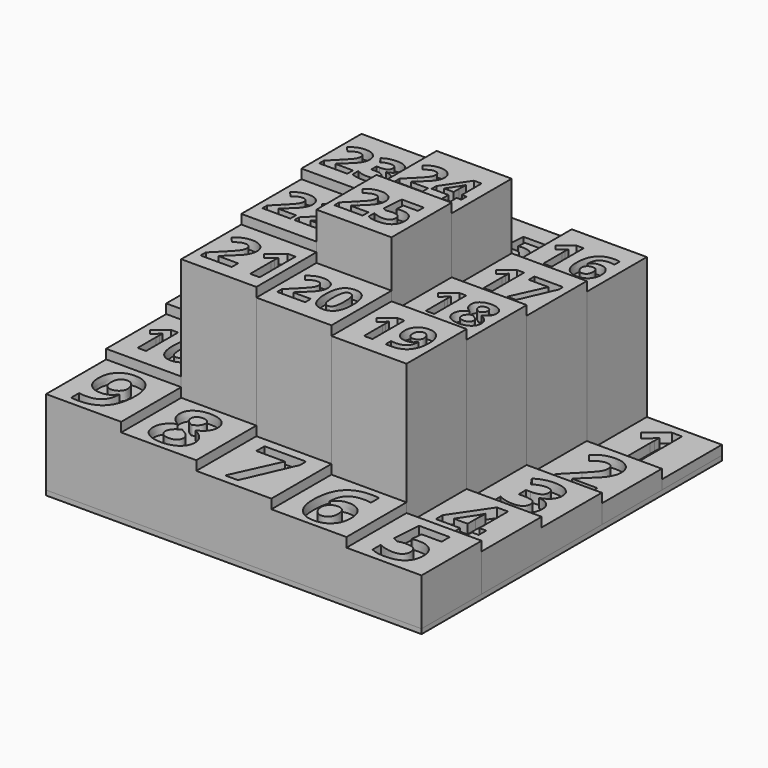
from build123d import *

# Parameters (mm, degrees)
F0_W          = 40
F0_H          = 40
F1_DEPTH      = 5
F2_W          = 40
F2_H          = 40
F3_DEPTH      = 10
F4_W          = 40
F4_H          = 40
F5_DEPTH      = 15
F6_W          = 40
F6_H          = 40
F7_DEPTH      = 20
F8_W          = 40
F8_H          = 40
F9_DEPTH      = 25
F10_W         = 40
F10_H         = 40
F11_DEPTH     = 30
F12_W         = 40
F12_H         = 40
F13_DEPTH     = 35
F14_W         = 40
F14_H         = 40
F15_DEPTH     = 40
F16_W         = 40
F16_H         = 40
F17_DEPTH     = 45
F18_W         = 40
F18_H         = 40
F19_DEPTH     = 50
F20_W         = 40
F20_H         = 40
F21_DEPTH     = 55
F22_W         = 40
F22_H         = 40
F23_DEPTH     = 60
F24_W         = 40
F24_H         = 40
F25_DEPTH     = 65
F26_W         = 40
F26_H         = 40
F27_DEPTH     = 70
F28_W         = 40
F28_H         = 40
F29_DEPTH     = 75
F30_W         = 40
F30_H         = 40
F31_DEPTH     = 80
F32_W         = 40
F32_H         = 40
F33_DEPTH     = 85
F34_W         = 40
F34_H         = 40
F35_DEPTH     = 90
F36_W         = 40
F36_H         = 40
F37_DEPTH     = 95
F38_W         = 40
F38_H         = 40
F39_DEPTH     = 100
F40_W         = 40
F40_H         = 40
F41_DEPTH     = 105
F42_W         = 40
F42_H         = 40
F43_DEPTH     = 110
F44_W         = 40
F44_H         = 40
F45_DEPTH     = 115
F46_W         = 40
F46_H         = 40
F47_DEPTH     = 120
F48_W         = 40
F48_H         = 40
F49_DEPTH     = 125
F50_TEXT_SIZE = 43.9635064039
F51_DEPTH     = 25.4
F52_TEXT_SIZE = 42.8115716204
F53_DEPTH     = 5
F54_TEXT_SIZE = 41.7113808605
F55_DEPTH     = 5
F56_TEXT_SIZE = 42.539030417
F57_DEPTH     = 5
F58_TEXT_SIZE = 42.0912582841
F59_DEPTH     = 5
F60_TEXT_SIZE = 45.2257071932
F61_DEPTH     = 5
F62_TEXT_SIZE = 43.1709095008
F63_DEPTH     = 5
F64_TEXT_SIZE = 44.5941256152
F65_DEPTH     = 5
F66_TEXT_SIZE = 44.0766827928
F67_DEPTH     = 5
F68_TEXT_SIZE = 29.8945682637
F69_DEPTH     = 5
F70_TEXT_SIZE = 33.3730631704
F71_DEPTH     = 5
F72_TEXT_SIZE = 29.7951582868
F73_DEPTH     = 5
F74_TEXT_SIZE = 29.970564624
F75_DEPTH     = 5
F76_TEXT_SIZE = 29.39246818
F77_DEPTH     = 5
F78_TEXT_SIZE = 30.131826742
F79_DEPTH     = 5
F80_TEXT_SIZE = 29.7951582868
F81_DEPTH     = 5
F82_TEXT_SIZE = 29.7951582868
F83_DEPTH     = 5
F84_TEXT_SIZE = 29.8706494199
F85_DEPTH     = 5
F86_TEXT_SIZE = 29.8706494199
F87_DEPTH     = 5
F88_TEXT_SIZE = 29.8945682637
F89_DEPTH     = 5
F90_TEXT_SIZE = 33.3730631704
F91_DEPTH     = 5
F92_TEXT_SIZE = 29.7951582868
F93_DEPTH     = 5
F94_TEXT_SIZE = 29.970564624
F95_DEPTH     = 5
F96_TEXT_SIZE = 29.39246818
F97_DEPTH     = 5
F98_TEXT_SIZE = 30.131826742
F99_DEPTH     = 5
F101_ANGLE    = 180
F102_W        = 200
F102_H        = 200
F103_DEPTH    = 2.54


# Not quite as in the source:
# - Text() gives the source's letters only with a copy of the font that has no kerning and outlines rounded to 1/6400 em; it was checked with that copy


with BuildPart() as f1:
    # F0 (on Top) → F1 (new body)
    with BuildSketch(Plane.XY):
        with Locations((-146.1425478756, 78.8295151293)):
            Rectangle(F0_W, F0_H)
    extrude(amount=F1_DEPTH)

    # F50 (on face) → F51 (cut)
    with BuildSketch(Plane.XY.offset(5)):
        with Locations((-161.8985384703, 62.9098713398)):
            Text('1', F50_TEXT_SIZE, font='Open Sans', font_style=FontStyle.BOLD, text_align=(TextAlign.LEFT, TextAlign.BOTTOM))
    extrude(amount=-F51_DEPTH, mode=Mode.SUBTRACT)


with BuildPart() as f3:
    # F2 (on face) → F3 (new body)
    with BuildSketch(Plane(origin=(0, 0, 0), x_dir=(1, 0, 0), z_dir=(0, 0, -1))):
        with Locations((-146.1425478756, -38.8295151293)):
            Rectangle(F2_W, F2_H)
    extrude(amount=-F3_DEPTH)

    # F52 (on face) → F53 (cut)
    with BuildSketch(Plane.XY.offset(10)):
        with Locations((-159.3360304832, 23.0267103761)):
            Text('2', F52_TEXT_SIZE, font='Open Sans', font_style=FontStyle.BOLD, text_align=(TextAlign.LEFT, TextAlign.BOTTOM))
    extrude(amount=-F53_DEPTH, mode=Mode.SUBTRACT)


with BuildPart() as f5:
    # F4 (on face) → F5 (new body)
    with BuildSketch(Plane(origin=(0, 0, 0), x_dir=(1, 0, 0), z_dir=(0, 0, -1))):
        with Locations((-146.1425478756, 1.1704848707)):
            Rectangle(F4_W, F4_H)
    extrude(amount=-F5_DEPTH)

    # F6 (on face) → F7 (join)
    with BuildSketch(Plane(origin=(0, 0, 0), x_dir=(1, 0, 0), z_dir=(0, 0, -1))):
        with Locations((-146.1425478756, 41.1704848707)):
            Rectangle(F6_W, F6_H)
    extrude(amount=-F7_DEPTH)

    # F54 (on face) → F55 (cut)
    with BuildSketch(Plane.XY.offset(15)):
        with Locations((-158.4442704916, -16.6733469814)):
            Text('3', F54_TEXT_SIZE, font='Open Sans', font_style=FontStyle.BOLD, text_align=(TextAlign.LEFT, TextAlign.BOTTOM))
    extrude(amount=-F55_DEPTH, mode=Mode.SUBTRACT)

    # F56 (on face) → F57 (cut)
    with BuildSketch(Plane.XY.offset(20)):
        with Locations((-159.9645316601, -56.619418785)):
            Text('4', F56_TEXT_SIZE, font='Open Sans', font_style=FontStyle.BOLD, text_align=(TextAlign.LEFT, TextAlign.BOTTOM))
    extrude(amount=-F57_DEPTH, mode=Mode.SUBTRACT)


with BuildPart() as f9:
    # F8 (on face) → F9 (new body)
    with BuildSketch(Plane(origin=(0, 0, 0), x_dir=(1, 0, 0), z_dir=(0, 0, -1))):
        with Locations((-146.1425478756, 81.1704848707)):
            Rectangle(F8_W, F8_H)
    extrude(amount=-F9_DEPTH)

    # F10 (on face) → F11 (join)
    with BuildSketch(Plane(origin=(0, 0, 0), x_dir=(1, 0, 0), z_dir=(0, 0, -1))):
        with Locations((-186.1425478756, 81.1704848707)):
            Rectangle(F10_W, F10_H)
    extrude(amount=-F11_DEPTH)

    # F12 (on face) → F13 (join)
    with BuildSketch(Plane(origin=(0, 0, 0), x_dir=(1, 0, 0), z_dir=(0, 0, -1))):
        with Locations((-226.1425478756, 81.1704848707)):
            Rectangle(F12_W, F12_H)
    extrude(amount=-F13_DEPTH)

    # F14 (on face) → F15 (join)
    with BuildSketch(Plane(origin=(0, 0, 0), x_dir=(1, 0, 0), z_dir=(0, 0, -1))):
        with Locations((-266.1425478756, 81.1704848707)):
            Rectangle(F14_W, F14_H)
    extrude(amount=-F15_DEPTH)

    # F16 (on face) → F17 (join)
    with BuildSketch(Plane(origin=(0, 0, 0), x_dir=(1, 0, 0), z_dir=(0, 0, -1))):
        with Locations((-306.1425478756, 81.1704848707)):
            Rectangle(F16_W, F16_H)
    extrude(amount=-F17_DEPTH)

    # F18 (on face) → F19 (join)
    with BuildSketch(Plane(origin=(0, 0, 0), x_dir=(1, 0, 0), z_dir=(0, 0, -1))):
        with Locations((-306.1425478756, 41.1704848707)):
            Rectangle(F18_W, F18_H)
    extrude(amount=-F19_DEPTH)

    # F20 (on face) → F21 (join)
    with BuildSketch(Plane(origin=(0, 0, 0), x_dir=(1, 0, 0), z_dir=(0, 0, -1))):
        with Locations((-306.1425478756, 1.1704848707)):
            Rectangle(F20_W, F20_H)
    extrude(amount=-F21_DEPTH)

    # F22 (on face) → F23 (join)
    with BuildSketch(Plane(origin=(0, 0, 0), x_dir=(1, 0, 0), z_dir=(0, 0, -1))):
        with Locations((-306.1425478756, -38.8295151293)):
            Rectangle(F22_W, F22_H)
    extrude(amount=-F23_DEPTH)

    # F58 (on face) → F59 (cut)
    with BuildSketch(Plane.XY.offset(25)):
        with Locations((-158.6749255657, -96.9195589423)):
            Text('5', F58_TEXT_SIZE, font='Open Sans', font_style=FontStyle.BOLD, text_align=(TextAlign.LEFT, TextAlign.BOTTOM))
    extrude(amount=-F59_DEPTH, mode=Mode.SUBTRACT)

    # F60 (on face) → F61 (cut)
    with BuildSketch(Plane.XY.offset(30)):
        with Locations((-199.6198743582, -97.5643545389)):
            Text('6', F60_TEXT_SIZE, font='Open Sans', font_style=FontStyle.BOLD, text_align=(TextAlign.LEFT, TextAlign.BOTTOM))
    extrude(amount=-F61_DEPTH, mode=Mode.SUBTRACT)

    # F62 (on face) → F63 (cut)
    with BuildSketch(Plane.XY.offset(35)):
        with Locations((-239.0029877424, -96.8608111143)):
            Text('7', F62_TEXT_SIZE, font='Open Sans', font_style=FontStyle.BOLD, text_align=(TextAlign.LEFT, TextAlign.BOTTOM))
    extrude(amount=-F63_DEPTH, mode=Mode.SUBTRACT)

    # F64 (on face) → F65 (cut)
    with BuildSketch(Plane.XY.offset(40)):
        with Locations((-280.3331911564, -97.2023829818)):
            Text('8', F64_TEXT_SIZE, font='Open Sans', font_style=FontStyle.BOLD, text_align=(TextAlign.LEFT, TextAlign.BOTTOM))
    extrude(amount=-F65_DEPTH, mode=Mode.SUBTRACT)

    # F66 (on face) → F67 (cut)
    with BuildSketch(Plane.XY.offset(45)):
        with Locations((-319.6105360985, -97.0161855221)):
            Text('9', F66_TEXT_SIZE, font='Open Sans', font_style=FontStyle.BOLD, text_align=(TextAlign.LEFT, TextAlign.BOTTOM))
    extrude(amount=-F67_DEPTH, mode=Mode.SUBTRACT)

    # F68 (on face) → F69 (cut)
    with BuildSketch(Plane.XY.offset(50)):
        with Locations((-324.2531219047, -52.3943256904)):
            Text('10', F68_TEXT_SIZE, font='Open Sans', font_style=FontStyle.BOLD, text_align=(TextAlign.LEFT, TextAlign.BOTTOM))
    extrude(amount=-F69_DEPTH, mode=Mode.SUBTRACT)

    # F70 (on face) → F71 (cut)
    with BuildSketch(Plane.XY.offset(55)):
        with Locations((-323.840325339, -13.2019839741)):
            Text('11', F70_TEXT_SIZE, font='Open Sans', font_style=FontStyle.BOLD, text_align=(TextAlign.LEFT, TextAlign.BOTTOM))
    extrude(amount=-F71_DEPTH, mode=Mode.SUBTRACT)

    # F72 (on face) → F73 (cut)
    with BuildSketch(Plane.XY.offset(60)):
        with Locations((-324.2819103489, 26.9366578012)):
            Text('12', F72_TEXT_SIZE, font='Open Sans', font_style=FontStyle.BOLD, text_align=(TextAlign.LEFT, TextAlign.BOTTOM))
    extrude(amount=-F73_DEPTH, mode=Mode.SUBTRACT)


with BuildPart() as f25:
    # F24 (on face) → F25 (new body)
    with BuildSketch(Plane(origin=(0, 0, 0), x_dir=(1, 0, 0), z_dir=(0, 0, -1))):
        with Locations((-306.1425478756, -78.8295151293)):
            Rectangle(F24_W, F24_H)
    extrude(amount=-F25_DEPTH)

    # F26 (on face) → F27 (join)
    with BuildSketch(Plane(origin=(0, 0, 0), x_dir=(1, 0, 0), z_dir=(0, 0, -1))):
        with Locations((-266.1425478756, -78.8295151293)):
            Rectangle(F26_W, F26_H)
    extrude(amount=-F27_DEPTH)

    # F74 (on face) → F75 (cut)
    with BuildSketch(Plane.XY.offset(65)):
        with Locations((-323.570565288, 67.1331060173)):
            Text('13', F74_TEXT_SIZE, font='Open Sans', font_style=FontStyle.BOLD, text_align=(TextAlign.LEFT, TextAlign.BOTTOM))
    extrude(amount=-F75_DEPTH, mode=Mode.SUBTRACT)

    # F76 (on face) → F77 (cut)
    with BuildSketch(Plane.XY.offset(70)):
        with Locations((-283.8859129857, 67.584938816)):
            Text('14', F76_TEXT_SIZE, font='Open Sans', font_style=FontStyle.BOLD, text_align=(TextAlign.LEFT, TextAlign.BOTTOM))
    extrude(amount=-F77_DEPTH, mode=Mode.SUBTRACT)


with BuildPart() as f29:
    # F28 (on face) → F29 (new body)
    with BuildSketch(Plane(origin=(0, 0, 0), x_dir=(1, 0, 0), z_dir=(0, 0, -1))):
        with Locations((-226.1425478756, -78.8295151293)):
            Rectangle(F28_W, F28_H)
    extrude(amount=-F29_DEPTH)

    # F78 (on face) → F79 (cut)
    with BuildSketch(Plane.XY.offset(75)):
        with Locations((-243.567291904, 67.0035963744)):
            Text('15', F78_TEXT_SIZE, font='Open Sans', font_style=FontStyle.BOLD, text_align=(TextAlign.LEFT, TextAlign.BOTTOM))
    extrude(amount=-F79_DEPTH, mode=Mode.SUBTRACT)


with BuildPart() as f31:
    # F30 (on face) → F31 (new body)
    with BuildSketch(Plane(origin=(0, 0, 0), x_dir=(1, 0, 0), z_dir=(0, 0, -1))):
        with Locations((-186.1425478756, -78.8295151293)):
            Rectangle(F30_W, F30_H)
    extrude(amount=-F31_DEPTH)

    # F80 (on face) → F81 (cut)
    with BuildSketch(Plane.XY.offset(80)):
        with Locations((-203.9077669813, 67.3344114036)):
            Text('16', F80_TEXT_SIZE, font='Open Sans', font_style=FontStyle.BOLD, text_align=(TextAlign.LEFT, TextAlign.BOTTOM))
    extrude(amount=-F81_DEPTH, mode=Mode.SUBTRACT)


with BuildPart() as f33:
    # F32 (on face) → F33 (new body)
    with BuildSketch(Plane(origin=(0, 0, 0), x_dir=(1, 0, 0), z_dir=(0, 0, -1))):
        with Locations((-186.1425478756, -38.8295151293)):
            Rectangle(F32_W, F32_H)
    extrude(amount=-F33_DEPTH)

    # F82 (on face) → F83 (cut)
    with BuildSketch(Plane.XY.offset(85)):
        with Locations((-203.5129799515, 27.1933717301)):
            Text('17', F82_TEXT_SIZE, font='Open Sans', font_style=FontStyle.BOLD, text_align=(TextAlign.LEFT, TextAlign.BOTTOM))
    extrude(amount=-F83_DEPTH, mode=Mode.SUBTRACT)


with BuildPart() as f35:
    # F34 (on face) → F35 (new body)
    with BuildSketch(Plane(origin=(0, 0, 0), x_dir=(1, 0, 0), z_dir=(0, 0, -1))):
        with Locations((-186.1425478756, 1.1704848707)):
            Rectangle(F34_W, F34_H)
    extrude(amount=-F35_DEPTH)

    # F84 (on face) → F85 (cut)
    with BuildSketch(Plane.XY.offset(90)):
        with Locations((-203.4901118982, -11.471883155)):
            Text('18', F84_TEXT_SIZE, font='Open Sans', font_style=FontStyle.BOLD, text_align=(TextAlign.LEFT, TextAlign.BOTTOM))
    extrude(amount=-F85_DEPTH, mode=Mode.SUBTRACT)


with BuildPart() as f37:
    # F36 (on face) → F37 (new body)
    with BuildSketch(Plane(origin=(0, 0, 0), x_dir=(1, 0, 0), z_dir=(0, 0, -1))):
        with Locations((-186.1425478756, 41.1704848707)):
            Rectangle(F36_W, F36_H)
    extrude(amount=-F37_DEPTH)

    # F86 (on face) → F87 (cut)
    with BuildSketch(Plane.XY.offset(95)):
        with Locations((-203.4383152363, -52.6618594744)):
            Text('19', F86_TEXT_SIZE, font='Open Sans', font_style=FontStyle.BOLD, text_align=(TextAlign.LEFT, TextAlign.BOTTOM))
    extrude(amount=-F87_DEPTH, mode=Mode.SUBTRACT)


with BuildPart() as f39:
    # F38 (on face) → F39 (new body)
    with BuildSketch(Plane(origin=(0, 0, 0), x_dir=(1, 0, 0), z_dir=(0, 0, -1))):
        with Locations((-226.1425478756, 41.1704848707)):
            Rectangle(F38_W, F38_H)
    extrude(amount=-F39_DEPTH)

    # F88 (on face) → F89 (cut)
    with BuildSketch(Plane.XY.offset(100)):
        with Locations((-243.8220114889, -51.7340404507)):
            Text('20', F88_TEXT_SIZE, font='Open Sans', font_style=FontStyle.BOLD, text_align=(TextAlign.LEFT, TextAlign.BOTTOM))
    extrude(amount=-F89_DEPTH, mode=Mode.SUBTRACT)


with BuildPart() as f41:
    # F40 (on face) → F41 (new body)
    with BuildSketch(Plane(origin=(0, 0, 0), x_dir=(1, 0, 0), z_dir=(0, 0, -1))):
        with Locations((-266.1425478756, 41.1704848707)):
            Rectangle(F40_W, F40_H)
    extrude(amount=-F41_DEPTH)

    # F90 (on face) → F91 (cut)
    with BuildSketch(Plane.XY.offset(105)):
        with Locations((-283.3203628548, -53.5402236553)):
            Text('21', F90_TEXT_SIZE, font='Open Sans', font_style=FontStyle.BOLD, text_align=(TextAlign.LEFT, TextAlign.BOTTOM))
    extrude(amount=-F91_DEPTH, mode=Mode.SUBTRACT)


with BuildPart() as f43:
    # F42 (on face) → F43 (new body)
    with BuildSketch(Plane(origin=(0, 0, 0), x_dir=(1, 0, 0), z_dir=(0, 0, -1))):
        with Locations((-266.1425478756, 1.1704848707)):
            Rectangle(F42_W, F42_H)
    extrude(amount=-F43_DEPTH)

    # F92 (on face) → F93 (cut)
    with BuildSketch(Plane.XY.offset(110)):
        with Locations((-283.6582310562, -11.7253012178)):
            Text('22', F92_TEXT_SIZE, font='Open Sans', font_style=FontStyle.BOLD, text_align=(TextAlign.LEFT, TextAlign.BOTTOM))
    extrude(amount=-F93_DEPTH, mode=Mode.SUBTRACT)


with BuildPart() as f45:
    # F44 (on face) → F45 (new body)
    with BuildSketch(Plane(origin=(0, 0, 0), x_dir=(1, 0, 0), z_dir=(0, 0, -1))):
        with Locations((-266.1425478756, -38.8295151293)):
            Rectangle(F44_W, F44_H)
    extrude(amount=-F45_DEPTH)

    # F94 (on face) → F95 (cut)
    with BuildSketch(Plane.XY.offset(115)):
        with Locations((-284.4813337052, 27.1075663503)):
            Text('23', F94_TEXT_SIZE, font='Open Sans', font_style=FontStyle.BOLD, text_align=(TextAlign.LEFT, TextAlign.BOTTOM))
    extrude(amount=-F95_DEPTH, mode=Mode.SUBTRACT)


with BuildPart() as f47:
    # F46 (on face) → F47 (new body)
    with BuildSketch(Plane(origin=(0, 0, 0), x_dir=(1, 0, 0), z_dir=(0, 0, -1))):
        with Locations((-226.1425478756, -38.8295151293)):
            Rectangle(F46_W, F46_H)
    extrude(amount=-F47_DEPTH)

    # F96 (on face) → F97 (cut)
    with BuildSketch(Plane.XY.offset(120)):
        with Locations((-243.7350419265, 26.6086359017)):
            Text('24', F96_TEXT_SIZE, font='Open Sans', font_style=FontStyle.BOLD, text_align=(TextAlign.LEFT, TextAlign.BOTTOM))
    extrude(amount=-F97_DEPTH, mode=Mode.SUBTRACT)


with BuildPart() as f49:
    # F48 (on face) → F49 (new body)
    with BuildSketch(Plane(origin=(0, 0, 0), x_dir=(1, 0, 0), z_dir=(0, 0, -1))):
        with Locations((-226.1425478756, 1.1704848707)):
            Rectangle(F48_W, F48_H)
    extrude(amount=-F49_DEPTH)

    # F98 (on face) → F99 (cut)
    with BuildSketch(Plane.XY.offset(125)):
        with Locations((-244.0136139392, -13.3618008085)):
            Text('25', F98_TEXT_SIZE, font='Open Sans', font_style=FontStyle.BOLD, text_align=(TextAlign.LEFT, TextAlign.BOTTOM))
    extrude(amount=-F99_DEPTH, mode=Mode.SUBTRACT)


with BuildPart() as f101_tool:
    # F100 (on face) → F101 (revolve)
    with BuildSketch(Plane(origin=(0, 0, 0), x_dir=(1, 0, 0), z_dir=(0, 0, -1))):
        with BuildLine():
            Line((-225.389104759, 21.1704848707), (-225.389104759, 57.2701077139))
            ThreePointArc((-225.389104759, 57.2701077139), (-282.2472300304, 1.1704848707), (-225.389104759, -54.9291379726))
            Line((-225.389104759, -54.9291379726), (-225.389104759, -18.8295151293))
            Line((-225.389104759, -18.8295151293), (-246.1425478756, -18.8295151293))
            Line((-246.1425478756, -18.8295151293), (-246.1425478756, 21.1704848707))
            Line((-246.1425478756, 21.1704848707), (-225.389104759, 21.1704848707))
        make_face()
    revolve(axis=Axis((-225.389104759, -1.1704848707, 0), (0, 1, 0)), revolution_arc=F101_ANGLE)


with BuildPart() as f33_1:
    add(f33.part)

    # F101: cut by f101_tool
    add(f101_tool.part, mode=Mode.SUBTRACT)


with BuildPart() as f35_1:
    add(f35.part)

    # F101: cut by f101_tool
    add(f101_tool.part, mode=Mode.SUBTRACT)


with BuildPart() as f37_1:
    add(f37.part)

    # F101: cut by f101_tool
    add(f101_tool.part, mode=Mode.SUBTRACT)


with BuildPart() as f39_1:
    add(f39.part)

    # F101: cut by f101_tool
    add(f101_tool.part, mode=Mode.SUBTRACT)


with BuildPart() as f41_1:
    add(f41.part)

    # F101: cut by f101_tool
    add(f101_tool.part, mode=Mode.SUBTRACT)


with BuildPart() as f43_1:
    add(f43.part)

    # F101: cut by f101_tool
    add(f101_tool.part, mode=Mode.SUBTRACT)


with BuildPart() as f45_1:
    add(f45.part)

    # F101: cut by f101_tool
    add(f101_tool.part, mode=Mode.SUBTRACT)


with BuildPart() as f47_1:
    add(f47.part)

    # F101: cut by f101_tool
    add(f101_tool.part, mode=Mode.SUBTRACT)


with BuildPart() as f103:
    # F102 (on face) → F103 (new body)
    with BuildSketch(Plane(origin=(0, 0, 0), x_dir=(1, 0, 0), z_dir=(0, 0, -1))):
        with Locations((-226.1425478756, 1.1704848707)):
            Rectangle(F102_W, F102_H)
    extrude(amount=F103_DEPTH)


solid = Compound([f1.part, f3.part, f5.part, f9.part, f25.part, f29.part, f31.part, f49.part, f33_1.part, f35_1.part, f37_1.part, f39_1.part, f41_1.part, f43_1.part, f45_1.part, f47_1.part, f103.part])
